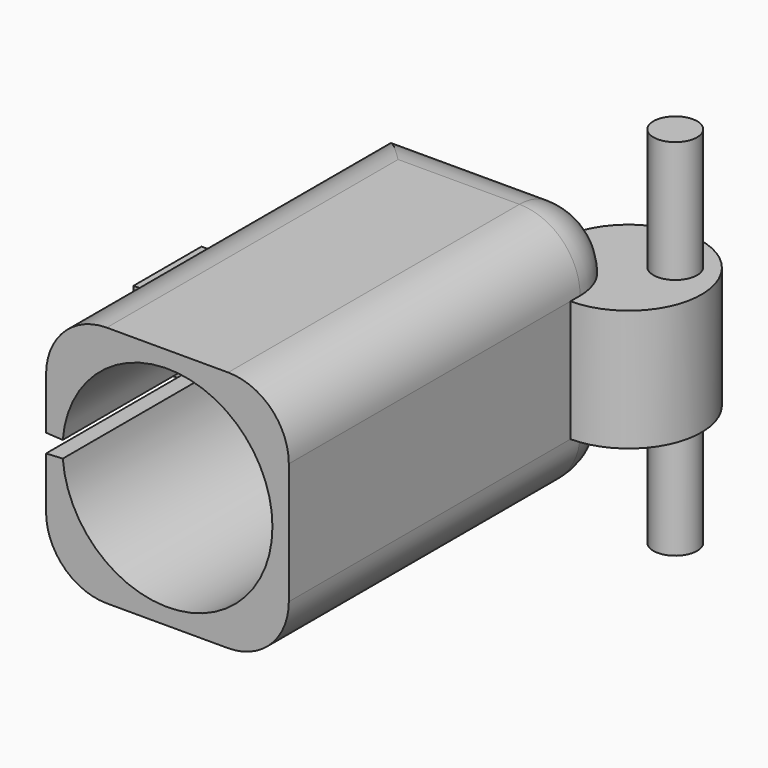
from build123d import *

# Parameters (mm, degrees)
F0_W      = 20
F0_H      = 20
F0_R      = 8.65
F1_DEPTH  = 20
F2_W      = 20
F2_H      = 20
F3_DEPTH  = 15
F4_R      = 4.75
F5_DEPTH  = 8
F6_R      = 2.075
F7_DEPTH  = 11
F9_DEPTH  = 25.3
F10_W     = 6
F10_H     = 2
F11_DEPTH = 3.5
F12_R     = 2.15
F13_DEPTH = 5.23
F14_R     = 1.65
F15_DEPTH = 6.34
F16_R     = 1.8
F17_DEPTH = 5
F18_R     = 5
F19_R     = 5
F20_R     = 4.99999
F21_R     = 3.5
F22_DEPTH = 31.8
F23_R     = 1.8
F24_DEPTH = 15


# Not quite as in the source:
# - a fillet or chamfer is up to 0.001 mm smaller than in the source, because OpenCascade refuses the exact size


with BuildPart() as f1:
    # F0 (on Front) → F1 (new body)
    with BuildSketch(Plane.XZ):
        Rectangle(F0_W, F0_H)
        Circle(F0_R, mode=Mode.SUBTRACT)
    extrude(amount=F1_DEPTH)

    # F2 (on Front) → F3 (join)
    with BuildSketch(Plane.XZ):
        Rectangle(F2_W, F2_H)
    extrude(amount=-F3_DEPTH)

    # F4 (on Front) → F5 (cut)
    with BuildSketch(Plane.XZ):
        Circle(F4_R)
    extrude(amount=-F5_DEPTH, mode=Mode.SUBTRACT)

    # F6 (on Front) → F7 (cut)
    with BuildSketch(Plane.XZ):
        Circle(F6_R)
    extrude(amount=-F7_DEPTH, mode=Mode.SUBTRACT)

    # F8 (on Front) → F9 (cut, symmetric)
    with BuildSketch(Plane.XZ):
        Polygon((4.25, 0), (-10, 0.75), (-10, -0.75), align=None)
    extrude(amount=F9_DEPTH, both=True, mode=Mode.SUBTRACT)

    # F10 (on Front) → F11 (join, symmetric)
    with BuildSketch(Plane.XZ):
        with Locations((-13, 1.75)):
            Rectangle(F10_W, F10_H)
        with Locations((-13, -1.75)):
            Rectangle(F10_W, F10_H)
    extrude(amount=F11_DEPTH, both=True)

    # F12 (on Top) → F13 (cut, symmetric)
    with BuildSketch(Plane.XY):
        with Locations((-13, 0)):
            Circle(F12_R)
    extrude(amount=F13_DEPTH, both=True, mode=Mode.SUBTRACT)

    # F14 (on Top) → F15 (cut)
    with BuildSketch(Plane.XY):
        with Locations((-13, 0)):
            Circle(F14_R)
    extrude(amount=-F15_DEPTH, mode=Mode.SUBTRACT)

    # F16 (on Top) → F17 (join, symmetric)
    with BuildSketch(Plane.XY):
        with BuildLine():
            Line((10, 15), (10, 9))
            ThreePointArc((10, 9), (14.2426406871, 19.2426406871), (4, 15))
            Line((4, 15), (10, 15))
        make_face()
        with Locations((12.2927147724, 16.93480205)):
            Circle(F16_R, mode=Mode.SUBTRACT)
    extrude(amount=F17_DEPTH, both=True)

    # F18
    f18_edges = [f1.edges().sort_by_distance(p)[0] for p in [
        (10, 15, 7.5),
    ]]
    fillet(f18_edges, radius=F18_R)

    # F19
    f19_edges = [f1.edges().sort_by_distance(p)[0] for p in [
        (10, 15, -7.5),
    ]]
    fillet(f19_edges, radius=F19_R)

    # F20 (radius 5 in the source; OpenCascade refuses exactly that, so slightly less here)
    f20_edges = [f1.edges().sort_by_distance(p)[0] for p in [
        (-10, -2.5, -10),
        (-10, -2.5, 10),
        (10, -5, -10),
        (10, -5, 10),
    ]]
    fillet(f20_edges, radius=F20_R)

    # F21 (on Front) → F22 (cut)
    with BuildSketch(Plane.XZ):
        Circle(F21_R)
    extrude(amount=-F22_DEPTH, mode=Mode.SUBTRACT)


with BuildPart() as f24:
    # F23 (on Top) → F24 (new body, symmetric)
    with BuildSketch(Plane.XY):
        with Locations((12.2927147724, 16.93480205)):
            Circle(F23_R)
    extrude(amount=F24_DEPTH, both=True)


solid = Compound([f1.part, f24.part])
